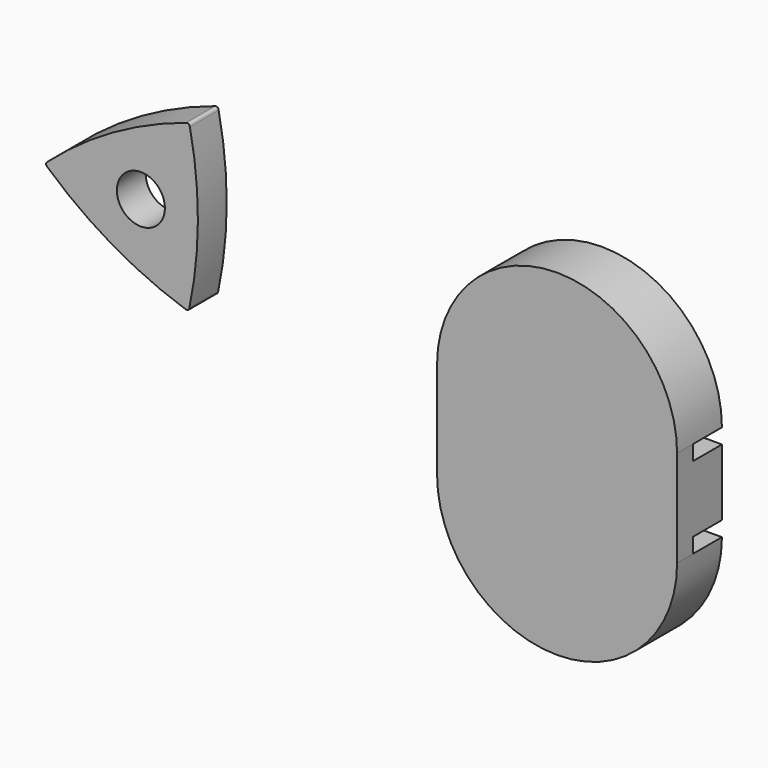
from build123d import *

# Parameters (mm, degrees)
F1_DEPTH    = 76.2
F2_R        = 12.7
F2_2_R      = 12.7
F4_DEPTH    = 42.3333333342
F5_R        = 50.8
F6_DEPTH    = 76.2
F7_T1_DEPTH = 111.4605556754


# Not quite as in the source:
# - a fillet or chamfer that OpenCascade refuses, or shapes differently, is made with other operations: its cross-section is extruded or revolved along the edge and cut away or added


with BuildPart() as f1:
    # F0 (on Front) → F1 (new body)
    with BuildSketch(Plane.XZ):
        with BuildLine():
            ThreePointArc((710.1282216017, -75.9319759618), (914.6043545827, 128.5441570192), (1119.0804875637, -75.9319759618))
            Line((1119.0804875637, -75.9319759618), (1168.6043545827, -75.9319759618))
            ThreePointArc((1168.6043545827, -75.9319759618), (914.6043545827, 178.0680240382), (660.6043545827, -75.9319759618))
            Line((660.6043545827, -75.9319759618), (710.1282216017, -75.9319759618))
        make_face()
    extrude(amount=F1_DEPTH)



with BuildPart() as f1b:
    # F0 (on Front) → F1, piece 2 (new body)
    with BuildSketch(Plane.XZ):
        with BuildLine():
            Line((1168.6043545827, -107.6819759618), (1116.6004596413, -107.6819759618))
            ThreePointArc((1116.6004596413, -107.6819759618), (1107.3920730747, -144.0743604042), (1091.6858802118, -178.1700424523))
            ThreePointArc((1091.6858802118, -178.1700424523), (1107.3920730747, -212.2657245004), (1116.6004596413, -248.6581089428))
            Line((1116.6004596413, -248.6581089428), (1168.6043545827, -248.6581089428))
            Line((1168.6043545827, -248.6581089428), (1168.6043545827, -107.6819759618))
        make_face()
    extrude(amount=F1_DEPTH)

    # F2#2
    f2_2_edges = [f1b.edges().sort_by_distance(p)[0] for p in [
        (1091.68588, -38.1, -178.170042),
    ]]
    fillet(f2_2_edges, radius=F2_2_R)


with BuildPart() as f1c:
    # F0 (on Front) → F1, piece 3 (new body)
    with BuildSketch(Plane.XZ):
        with BuildLine():
            ThreePointArc((737.5228289535, -178.1700424523), (727.8732059552, -159.2504438494), (720.2381050462, -139.4319759618))
            Line((720.2381050462, -139.4319759618), (660.6043545827, -139.4319759618))
            Line((660.6043545827, -139.4319759618), (660.6043545827, -216.9081089428))
            Line((660.6043545827, -216.9081089428), (720.2381050462, -216.9081089428))
            ThreePointArc((720.2381050462, -216.9081089428), (727.8732059552, -197.0896410552), (737.5228289535, -178.1700424523))
        make_face()
    extrude(amount=F1_DEPTH)

    # F2
    f2_edges = [f1c.edges().sort_by_distance(p)[0] for p in [
        (737.522829, -38.1, -178.170042),
    ]]
    fillet(f2_edges, radius=F2_R)


with BuildPart() as f1d:
    # F0 (on Front) → F1, piece 4 (new body)
    with BuildSketch(Plane.XZ):
        with BuildLine():
            Line((1168.6043545827, -280.4081089428), (1119.0804875637, -280.4081089428))
            ThreePointArc((1119.0804875637, -280.4081089428), (914.6043545827, -484.8842419238), (710.1282216017, -280.4081089428))
            Line((710.1282216017, -280.4081089428), (660.6043545827, -280.4081089428))
            ThreePointArc((660.6043545827, -280.4081089428), (914.6043545827, -534.4081089428), (1168.6043545827, -280.4081089428))
        make_face()
    extrude(amount=F1_DEPTH)


with BuildPart() as f1_1:
    add(f1.part)

    add(f1b.part)  # F4 merges F1b

    add(f1c.part)  # F4 merges F1c

    add(f1d.part)  # F4 merges F1d
    # F3 (on face) → F4 (join)
    with BuildSketch(Plane.XZ.offset(76.2)):
        with BuildLine():
            Line((1168.6043545827, -280.4081089428), (1168.6043545827, -75.9319759618))
            ThreePointArc((1168.6043545827, -75.9319759618), (914.6043545827, 178.0680240382), (660.6043545827, -75.9319759618))
            Line((660.6043545827, -75.9319759618), (660.6043545827, -280.4081089428))
            ThreePointArc((660.6043545827, -280.4081089428), (914.6043545827, -534.4081089428), (1168.6043545827, -280.4081089428))
        make_face()
    extrude(amount=F4_DEPTH)


with BuildPart() as f6:
    # F5 (on Front) → F6 (new body)
    with BuildSketch(Plane.XZ):
        with BuildLine():
            ThreePointArc((102.1237551128, 175.6729308734), (-60.0134851065, 104.6652000685), (-203.1990984501, 0.6053008208))
            Line((-203.1990984501, 0.6053008208), (102.1237551128, 175.6729308734))
        make_face()
        Polygon((102.1237551128, 175.6729308734), (-203.1990984501, 0.6053008208), (101.0753433373, -176.2782316942), align=None)
        Circle(F5_R, mode=Mode.SUBTRACT)
        with BuildLine():
            Line((101.0753433373, -176.2782316942), (-203.1990984501, 0.6053008208))
            ThreePointArc((-203.1990984501, 0.6053008208), (-60.6359795982, -104.3058027061), (101.0753433373, -176.2782316942))
        make_face()
        with BuildLine():
            ThreePointArc((101.0753433373, -176.2782316942), (120.6494647047, -0.3593973623), (102.1237551128, 175.6729308734))
            Line((102.1237551128, 175.6729308734), (101.0753433373, -176.2782316942))
        make_face()
    extrude(amount=F6_DEPTH)

    # F7: fillet of radius 6.35 on 3 edges, made by hand

    # F7_s2 → F7_t1 (cut)
    with BuildSketch(Plane.XZ.offset(-17.6302778377)):
        with BuildLine():
            add(Edge.make_bspline(
                [(95.406162744, 173.5267192743), (102.1465266623, 175.7121024143), (103.5827984, 168.7734045022)],
                knots=[0, 0, 0, 1, 1, 1], degree=2, weights=[1, 1, 1]))
            ThreePointArc((103.5827984, 168.7734045022), (102.8606729274, 172.2247317566), (102.1237551128, 175.6729308734))
            ThreePointArc((102.1237551128, 175.6729308734), (98.7626582273, 174.6070262148), (95.406162744, 173.5267192743))
        make_face()
        with BuildLine():
            add(Edge.make_bspline(
                [(94.3706565821, -174.0920370606), (101.097881112, -176.3175382051), (102.5754657549, -169.387520251)],
                knots=[0, 0, 0, 1, 1, 1], degree=2, weights=[1, 1, 1]))
            ThreePointArc((102.5754657549, -169.387520251), (101.8327912676, -172.8344840775), (101.0753433373, -176.2782316942))
            ThreePointArc((101.0753433373, -176.2782316942), (97.7206563975, -175.1923216837), (94.3706565821, -174.0920370606))
        make_face()
        with BuildLine():
            add(Edge.make_bspline(
                [(-197.9534549821, 5.3186325584), (-203.2444077743, 0.6054357907), (-197.9816284989, -4.1391990233)],
                knots=[0, 0, 0, 1, 1, 1], degree=2, weights=[1, 1, 1]))
            ThreePointArc((-197.9816284989, -4.1391990233), (-200.5954494949, -1.7725421373), (-203.1990984501, 0.6053008208))
            ThreePointArc((-203.1990984501, 0.6053008208), (-200.5813293248, 2.9675899272), (-197.9534549821, 5.3186325584))
        make_face()
    extrude(amount=F7_T1_DEPTH, mode=Mode.SUBTRACT)


solid = Compound([f1_1.part, f6.part])
